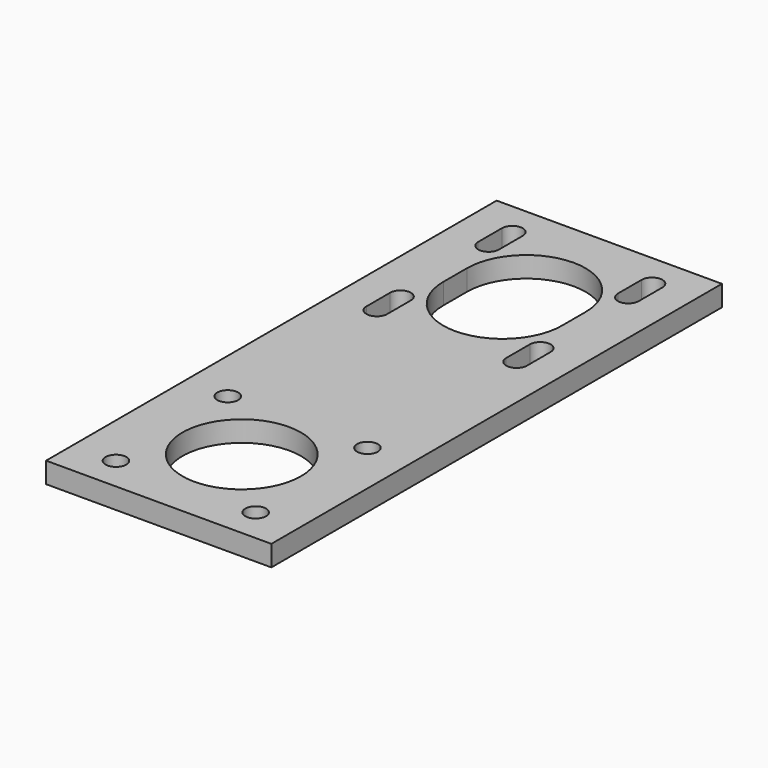
from build123d import *

# Parameters (mm, degrees)
F0_W     = 76
F0_H     = 190
F0_R     = 3.5
F0_R_2   = 20
F1_DEPTH = 7


# Not quite as in the source:
# - a feature names something its author has since deleted; it is built from what else it names


with BuildPart() as f1:
    # F0 (on Top) → F1 (new body)
    with BuildSketch(Plane.XY):
        with Locations((0, 60)):
            Rectangle(F0_W, F0_H)
        with Locations((-23.57, -23.57)):
            Circle(F0_R, mode=Mode.SUBTRACT)
        with Locations((-23.57, 23.57)):
            Circle(F0_R, mode=Mode.SUBTRACT)
        Circle(F0_R_2, mode=Mode.SUBTRACT)
        with Locations((23.57, -23.57)):
            Circle(F0_R, mode=Mode.SUBTRACT)
        with Locations((23.57, 23.57)):
            Circle(F0_R, mode=Mode.SUBTRACT)
        with BuildLine():
            Line((-27.07, 86.43), (-27.07, 96.43))
            ThreePointArc((-27.07, 96.43), (-23.5699996641, 99.93), (-20.07, 96.4299993282))
            Line((-20.07, 96.4299993282), (-20.07, 86.4299993282))
            ThreePointArc((-20.07, 86.4299993282), (-23.5700003359, 82.93), (-27.07, 86.43))
        make_face(mode=Mode.SUBTRACT)
        with BuildLine():
            Line((-27.07, 133.57), (-27.07, 143.57))
            ThreePointArc((-27.07, 143.57), (-23.5699996641, 147.07), (-20.07, 143.5699993282))
            Line((-20.07, 143.5699993282), (-20.07, 133.5699993282))
            ThreePointArc((-20.07, 133.5699993282), (-23.5700003359, 130.07), (-27.07, 133.57))
        make_face(mode=Mode.SUBTRACT)
        with BuildLine():
            Line((20.07, 86.43), (20.07, 96.43))
            ThreePointArc((20.07, 96.43), (23.5700003359, 99.93), (27.07, 96.4299993282))
            Line((27.07, 96.4299993282), (27.07, 86.4299993282))
            ThreePointArc((27.07, 86.4299993282), (23.5699996641, 82.93), (20.07, 86.43))
        make_face(mode=Mode.SUBTRACT)
        with BuildLine():
            Line((-20, 110), (-20, 120))
            ThreePointArc((-20, 120), (1.2657e-06, 140), (20, 119.9999974687))
            Line((20, 119.9999974687), (20, 109.9999974687))
            ThreePointArc((20, 109.9999974687), (-1.2657e-06, 90), (-20, 110))
        make_face(mode=Mode.SUBTRACT)
        with BuildLine():
            Line((20.07, 133.57), (20.07, 143.57))
            ThreePointArc((20.07, 143.57), (23.5700003359, 147.07), (27.07, 143.5699993282))
            Line((27.07, 143.5699993282), (27.07, 133.5699993282))
            ThreePointArc((27.07, 133.5699993282), (23.5699996641, 130.07), (20.07, 133.57))
        make_face(mode=Mode.SUBTRACT)
    extrude(amount=F1_DEPTH)


solid = f1.part
